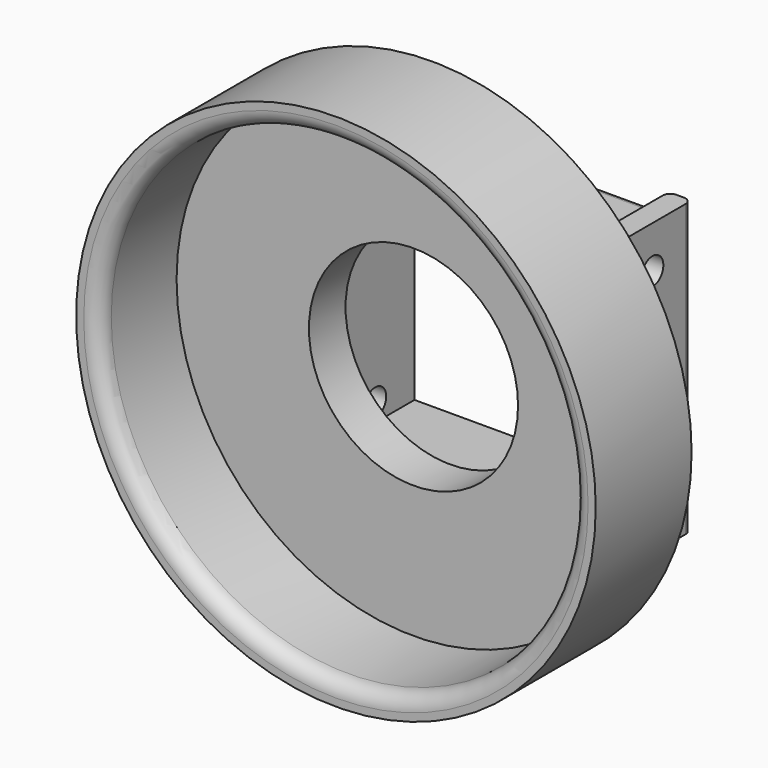
from build123d import *

# Parameters (mm, degrees)
F0_R     = 34.038
F0_R_2   = 31.038
F0_W     = 38.1
F0_H     = 38.1
F0_R_3   = 13.7
F1_DEPTH = 3
F2_DEPTH = 3
F3_DEPTH = 15.7
F4_R     = 2
F5_W     = 3
F5_H     = 38.1
F5_W_2   = 33.528
F5_H_2   = 33.528
F5_W_3   = 28.528
F5_H_3   = 31.528
F6_DEPTH = 15
F7_R     = 0.99999
F8_R     = 1.778
F9_DEPTH = 56.089


# Not quite as in the source:
# - a fillet or chamfer is up to 0.001 mm smaller than in the source, because OpenCascade refuses the exact size
# - a feature names something its author has since deleted; it is built from what else it names


with BuildPart() as f1:
    # F0 (on Front) → F1 (new body)
    with BuildSketch(Plane.XZ):
        Circle(F0_R)
        Circle(F0_R_2, mode=Mode.SUBTRACT)
        Circle(F0_R_2)
        Rectangle(F0_W, F0_H, mode=Mode.SUBTRACT)
        Rectangle(F0_W, F0_H)
        Circle(F0_R_3, mode=Mode.SUBTRACT)
    extrude(amount=F1_DEPTH)

    # F0 (on Front) → F2 (join)
    with BuildSketch(Plane.XZ):
        Rectangle(F0_W, F0_H)
        Circle(F0_R_3, mode=Mode.SUBTRACT)
    extrude(amount=-F2_DEPTH)

    # F0 (on Front) → F3 (join)
    with BuildSketch(Plane.XZ):
        Circle(F0_R)
        Circle(F0_R_2, mode=Mode.SUBTRACT)
    extrude(amount=F3_DEPTH)

    # F4
    f4_edges = [f1.edges().sort_by_distance(p)[0] for p in [
        (-31.038, -15.7, 0),
    ]]
    fillet(f4_edges, radius=F4_R)

    # F5 (on Front) → F6 (join)
    with BuildSketch(Plane.XZ):
        with Locations((-20.55, 0)):
            Rectangle(F5_W, F5_H)
        with Locations((20.55, 0)):
            Rectangle(F5_W, F5_H)
        Rectangle(F5_W_2, F5_H_2)
        Rectangle(F5_W_3, F5_H_3, mode=Mode.SUBTRACT)
    extrude(amount=-F6_DEPTH)

    # F7 (radius 1 in the source; OpenCascade refuses exactly that, so slightly less here)
    f7_edges = [f1.edges().sort_by_distance(p)[0] for p in [
        (-19.05, 15, 0),
        (-16.764, 15, 0),
        (19.05, 15, 0),
        (16.764, 15, 0),
        (0, 15, 16.764),
        (0, 15, -16.764),
        (22.05, 15, 0),
        (-22.05, 15, 0),
    ]]
    fillet(f7_edges, radius=F7_R)

    # F8 (on face) → F9 (cut, through all)
    with BuildSketch(Plane(origin=(-22.05, 0, 0), x_dir=(0, -1, 0), z_dir=(-1, 0, 0))):
        with Locations((-8.5796158184, 13.4703841816)):
            Circle(F8_R)
        with Locations((-8.5796158184, -13.4703841816)):
            Circle(F8_R)
    extrude(amount=-F9_DEPTH, mode=Mode.SUBTRACT)


solid = f1.part
